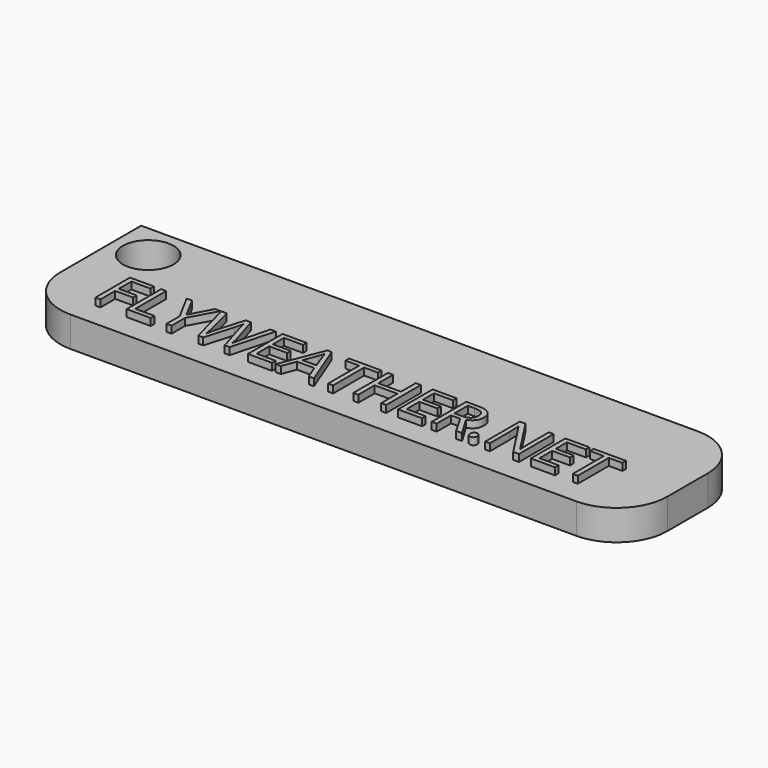
from build123d import *

# Parameters (mm, degrees)
F0_W         = 60
F0_H         = 15
F1_DEPTH     = 3
F2_R         = 5
F3_R         = 2.5
F4_DEPTH     = 25
F5_TEXT_SIZE = 5.980861244
F6_DEPTH     = 0.7


# Not quite as in the source:
# - Text() gives the source's letters only with a copy of the font that has no kerning and outlines rounded to 1/6400 em; it was checked with that copy


with BuildPart() as f1:
    # F0 (on Top) → F1 (new body)
    with BuildSketch(Plane.XY):
        with Locations((30, -7.5)):
            Rectangle(F0_W, F0_H)
    extrude(amount=F1_DEPTH)

    # F2
    f2_edges = [f1.edges().sort_by_distance(p)[0] for p in [
        (60, -15, 1.5),
        (60, 0, 1.5),
        (0, -15, 1.5),
    ]]
    fillet(f2_edges, radius=F2_R)

    # F3 (on face) → F4 (cut)
    with BuildSketch(Plane.XY.offset(3)):
        with Locations((3.5, -3.5)):
            Circle(F3_R)
    extrude(amount=-F4_DEPTH, mode=Mode.SUBTRACT)

    # F5 (on face) → F6 (join)
    with BuildSketch(Plane.XY.offset(3)):
        with Locations((5, -12.6359454845)):
            Text('FLYWEATHER.NET', F5_TEXT_SIZE, font='Open Sans', text_align=(TextAlign.LEFT, TextAlign.BOTTOM))
    extrude(amount=F6_DEPTH)


solid = f1.part
